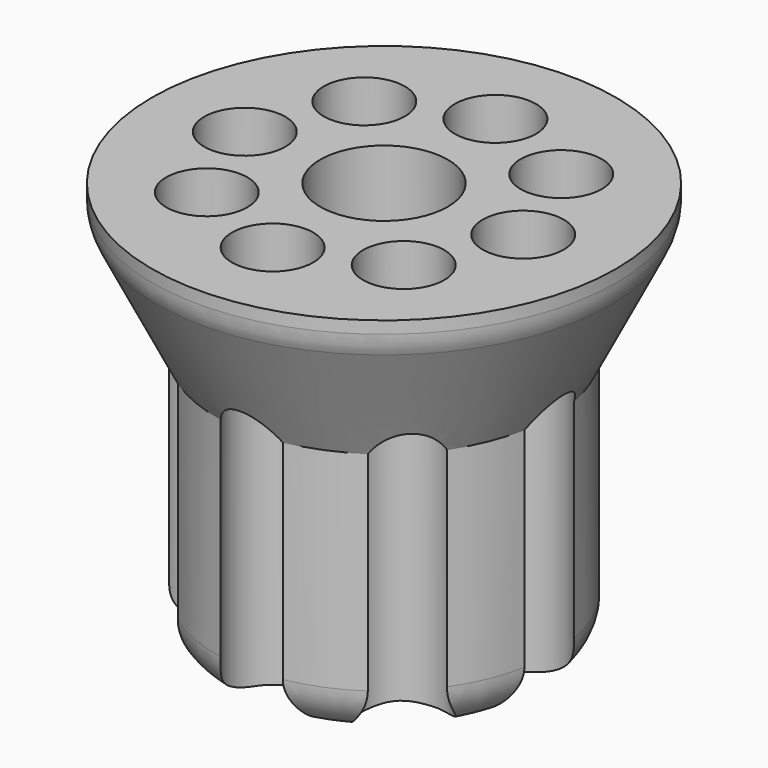
from build123d import *

# Parameters (mm, degrees)
F0_R         = 7.25
F1_DEPTH     = 10.5
F2_R         = 10
F3_DEPTH     = 7
F4_S5_R      = 7.25
F4_T6_DEPTH  = 16
F5_R         = 2.75
F6_DEPTH     = 25
F5_R_2       = 1.75
F7_DEPTH     = 25
F8_T2_ANGLE  = 102.7210494726
F8_T4_ANGLE  = 102.7210494726
F8_T6_ANGLE  = 102.7210494726
F8_T8_ANGLE  = 102.7210494726
F8_T10_ANGLE = 102.7210494726
F8_T12_ANGLE = 102.7210494726
F8_T14_ANGLE = 102.7210494726
F8_T16_ANGLE = 102.7210494726


# Not quite as in the source:
# - a fillet or chamfer that OpenCascade refuses, or shapes differently, is made with other operations: its cross-section is extruded or revolved along the edge and cut away or added


with BuildPart() as f1:
    # F0 (on Top) → F1 (new body)
    with BuildSketch(Plane.XY):
        Circle(F0_R)
    extrude(amount=-F1_DEPTH)

    # F2 (on Top) → F3 (join)
    with BuildSketch(Plane.XY):
        Circle(F2_R)
    extrude(amount=F3_DEPTH)

    # F4: chamfer of 6 x 3 on 1 edges, made by hand


with BuildPart() as f4_tool2:
    # F4_s3 → F4_t4 (revolve)
    with BuildSketch(Plane.XZ):
        Polygon((10, 6), (7, 0), (10, 0), align=None)
    revolve(axis=Axis((0, 0, 0), (0, 0, 1)))

    # F4_s5 → F4_t6 (cut, symmetric)
    with BuildSketch(Plane.XY.offset(3)):
        Circle(F4_S5_R)
    extrude(amount=F4_T6_DEPTH, both=True, mode=Mode.SUBTRACT)


with BuildPart() as f1_1:
    add(f1.part)

    # F4_t1: cut F4_tool2
    add(f4_tool2.part, mode=Mode.SUBTRACT)

    # F5 (on face) → F6 (cut)
    with BuildSketch(Plane.XY.offset(7)):
        Circle(F5_R)
    extrude(amount=-F6_DEPTH, mode=Mode.SUBTRACT)

    # F5 (on face) → F7 (cut)
    with BuildSketch(Plane.XY.offset(7)):
        with Locations((4.2426406871, 4.2426406871)):
            Circle(F5_R_2)
        with Locations((0, 6)):
            Circle(F5_R_2)
        with Locations((-4.2426406871, 4.2426406871)):
            Circle(F5_R_2)
        with Locations((-6, 0)):
            Circle(F5_R_2)
        with Locations((-4.2426406871, -4.2426406871)):
            Circle(F5_R_2)
        with Locations((6, 0)):
            Circle(F5_R_2)
        with Locations((0, -6)):
            Circle(F5_R_2)
        with Locations((4.2426406871, -4.2426406871)):
            Circle(F5_R_2)
    extrude(amount=-F7_DEPTH, mode=Mode.SUBTRACT)

    # F8: fillet of radius 2 on 10 edges, made by hand

    # F8_s1 → F8_t2 (revolve, cut)
    with BuildSketch(Plane(origin=(0, 0, 0), x_dir=(0, 0, 1), z_dir=(0.2779765386, -0.9605878637, 0))):
        with BuildLine():
            ThreePointArc((-8.5, -7.25), (-9.9142135624, -6.6642135624), (-10.5, -5.25))
            Line((-10.5, -5.25), (-10.5, -7.25))
            Line((-10.5, -7.25), (-8.5, -7.25))
        make_face()
    revolve(axis=Axis((0, 0, -10.5), (0, 0, 1)), revolution_arc=F8_T2_ANGLE, mode=Mode.SUBTRACT)

    # F8_s3 → F8_t4 (revolve, cut)
    with BuildSketch(Plane(origin=(0, 0, 0), x_dir=(0, 0, 1), z_dir=(-0.4826790969, -0.8757972879, 0))):
        with BuildLine():
            ThreePointArc((-8.5, -7.25), (-9.9142135624, -6.6642135624), (-10.5, -5.25))
            Line((-10.5, -5.25), (-10.5, -7.25))
            Line((-10.5, -7.25), (-8.5, -7.25))
        make_face()
    revolve(axis=Axis((0, 0, -10.5), (0, 0, 1)), revolution_arc=F8_T4_ANGLE, mode=Mode.SUBTRACT)

    # F8_s5 → F8_t6 (revolve, cut)
    with BuildSketch(Plane(origin=(0, 0, 0), x_dir=(0, 0, 1), z_dir=(0.8757972879, -0.4826790969, 0))):
        with BuildLine():
            ThreePointArc((-8.5, -7.25), (-9.9142135624, -6.6642135624), (-10.5, -5.25))
            Line((-10.5, -5.25), (-10.5, -7.25))
            Line((-10.5, -7.25), (-8.5, -7.25))
        make_face()
    revolve(axis=Axis((0, 0, -10.5), (0, 0, 1)), revolution_arc=F8_T6_ANGLE, mode=Mode.SUBTRACT)

    # F8_s7 → F8_t8 (revolve, cut)
    with BuildSketch(Plane(origin=(0, 0, 0), x_dir=(0, 0, 1), z_dir=(0.9605878637, 0.2779765386, 0))):
        with BuildLine():
            ThreePointArc((-8.5, -7.25), (-9.9142135624, -6.6642135624), (-10.5, -5.25))
            Line((-10.5, -5.25), (-10.5, -7.25))
            Line((-10.5, -7.25), (-8.5, -7.25))
        make_face()
    revolve(axis=Axis((0, 0, -10.5), (0, 0, 1)), revolution_arc=F8_T8_ANGLE, mode=Mode.SUBTRACT)

    # F8_s9 → F8_t10 (revolve, cut)
    with BuildSketch(Plane(origin=(0, 0, 0), x_dir=(0, 0, 1), z_dir=(0.4826790969, 0.8757972879, 0))):
        with BuildLine():
            ThreePointArc((-8.5, -7.25), (-9.9142135624, -6.6642135624), (-10.5, -5.25))
            Line((-10.5, -5.25), (-10.5, -7.25))
            Line((-10.5, -7.25), (-8.5, -7.25))
        make_face()
    revolve(axis=Axis((0, 0, -10.5), (0, 0, 1)), revolution_arc=F8_T10_ANGLE, mode=Mode.SUBTRACT)

    # F8_s11 → F8_t12 (revolve, cut)
    with BuildSketch(Plane(origin=(0, 0, 0), x_dir=(0, 0, 1), z_dir=(-0.2779765386, 0.9605878637, 0))):
        with BuildLine():
            ThreePointArc((-8.5, -7.25), (-9.9142135624, -6.6642135624), (-10.5, -5.25))
            Line((-10.5, -5.25), (-10.5, -7.25))
            Line((-10.5, -7.25), (-8.5, -7.25))
        make_face()
    revolve(axis=Axis((0, 0, -10.5), (0, 0, 1)), revolution_arc=F8_T12_ANGLE, mode=Mode.SUBTRACT)

    # F8_s13 → F8_t14 (revolve, cut)
    with BuildSketch(Plane(origin=(0, 0, 0), x_dir=(0, 0, 1), z_dir=(-0.8757972879, 0.4826790969, 0))):
        with BuildLine():
            ThreePointArc((-8.5, -7.25), (-9.9142135624, -6.6642135624), (-10.5, -5.25))
            Line((-10.5, -5.25), (-10.5, -7.25))
            Line((-10.5, -7.25), (-8.5, -7.25))
        make_face()
    revolve(axis=Axis((0, 0, -10.5), (0, 0, 1)), revolution_arc=F8_T14_ANGLE, mode=Mode.SUBTRACT)

    # F8_s15 → F8_t16 (revolve, cut)
    with BuildSketch(Plane(origin=(0, 0, 0), x_dir=(0, 0, 1), z_dir=(-0.9605878637, -0.2779765386, 0))):
        with BuildLine():
            ThreePointArc((-8.5, -7.25), (-9.9142135624, -6.6642135624), (-10.5, -5.25))
            Line((-10.5, -5.25), (-10.5, -7.25))
            Line((-10.5, -7.25), (-8.5, -7.25))
        make_face()
    revolve(axis=Axis((0, 0, -10.5), (0, 0, 1)), revolution_arc=F8_T16_ANGLE, mode=Mode.SUBTRACT)

    # F8_s17 → F8_t18 (revolve, cut)
    with BuildSketch(Plane.XZ):
        with BuildLine():
            ThreePointArc((2.75, -8.5), (3.3357864376, -9.9142135624), (4.75, -10.5))
            Line((4.75, -10.5), (2.75, -10.5))
            Line((2.75, -10.5), (2.75, -8.5))
        make_face()
    revolve(axis=Axis((0, 0, -10.5), (0, 0, 1)), mode=Mode.SUBTRACT)

    # F8_s19 → F8_t20 (revolve, cut)
    with BuildSketch(Plane.XZ):
        with BuildLine():
            ThreePointArc((10, 6.472135955), (9.9464979789, 6.0126301139), (9.788854382, 5.577708764))
            Line((9.788854382, 5.577708764), (10, 6))
            Line((10, 6), (10, 6.472135955))
        make_face()
    revolve(axis=Axis((0, 0, 6), (0, 0, 1)), mode=Mode.SUBTRACT)


solid = f1_1.part
